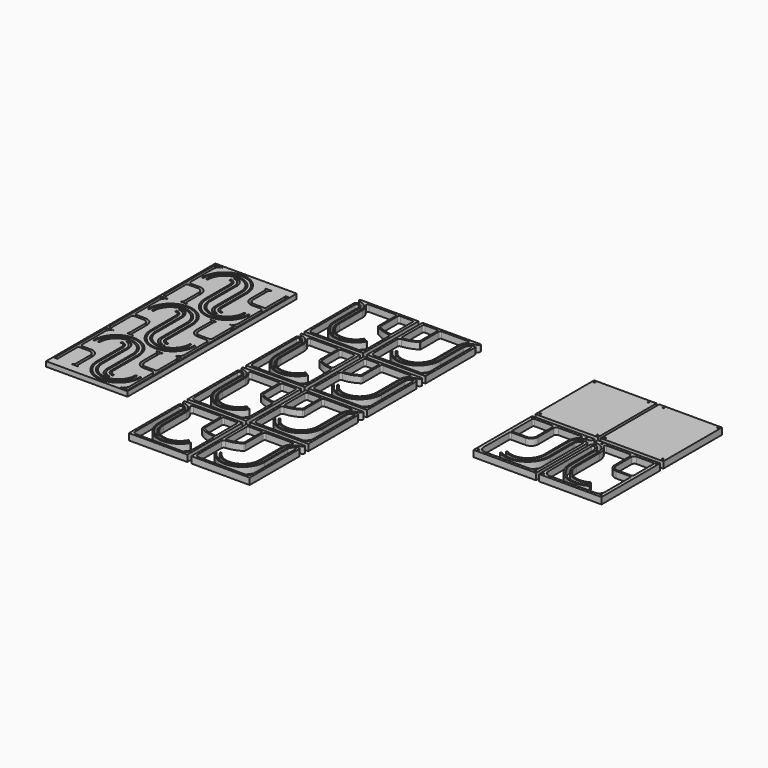
from build123d import *

# Parameters (mm, degrees)
F0_W     = 300
F0_H     = 780
F1_DEPTH = 18
F2_R     = 3
F3_DEPTH = 24
F2_W     = 230
F2_H     = 270
F2_W_2   = 231.0000000001
F5_DEPTH = 24


# Not quite as in the source:
# - a pattern or mirror of a feature is missing from the dataset's text; its kind, count and spacing are read off the source's solid


with BuildPart() as f1:
    # F0 (on Top) → F1 (new body)
    with BuildSketch(Plane.XY):
        with Locations((-546.0000000001, 50)):
            Rectangle(F0_W, F0_H)
        with BuildLine():
            Line((-690, -68), (-660, -68))
            ThreePointArc((-660, -68), (-674.1421356237, -73.8578643763), (-680, -88))
            Line((-680, -88), (-680, -192))
            ThreePointArc((-680, -192), (-677.0710678119, -199.0710678119), (-670, -202))
            Line((-670, -202), (-640, -202))
            ThreePointArc((-640, -202), (-618.7867965644, -210.7867965644), (-610, -232))
            Line((-610, -232), (-610, -298))
            ThreePointArc((-610, -298), (-607.0710678119, -305.0710678119), (-600, -308))
            Line((-600, -308), (-630, -308))
            ThreePointArc((-630, -308), (-622.9289321881, -305.0710678119), (-620, -298))
            Line((-620, -298), (-620, -232))
            ThreePointArc((-620, -232), (-625.8578643763, -217.8578643763), (-640, -212))
            Line((-640, -212), (-675, -212))
            ThreePointArc((-675, -212), (-678.5355339059, -213.4644660941), (-680, -217))
            Line((-680, -217), (-680, -303))
            ThreePointArc((-680, -303), (-678.5355339059, -306.5355339059), (-675, -308))
            Line((-675, -308), (-690, -308))
            Line((-690, -308), (-690, -68))
        make_face(mode=Mode.SUBTRACT)
        with BuildLine():
            ThreePointArc((-490, -290), (-506.9705627485, -282.9705627485), (-514, -266))
            Line((-514, -266), (-514, -150))
            ThreePointArc((-514, -150), (-590, -74), (-666, -150))
            ThreePointArc((-666, -150), (-669, -153), (-672, -150))
            ThreePointArc((-672, -150), (-590, -68), (-508, -150))
            Line((-508, -150), (-508, -266))
            ThreePointArc((-508, -266), (-502.7279220614, -278.7279220614), (-490, -284))
            Line((-490, -284), (-490, -290))
        make_face(mode=Mode.SUBTRACT)
        with BuildLine():
            ThreePointArc((-515, -300), (-526.6880815177, -284.8476830225), (-530, -266))
            Line((-530, -266), (-530, -150))
            ThreePointArc((-530, -150), (-590, -90), (-650, -150))
            ThreePointArc((-650, -150), (-653, -153), (-656, -150))
            ThreePointArc((-656, -150), (-590, -84), (-524, -150))
            Line((-524, -150), (-524, -266))
            ThreePointArc((-524, -266), (-514.0416305603, -290.0416305603), (-490, -300))
            Line((-490, -300), (-515, -300))
        make_face(mode=Mode.SUBTRACT)
        with BuildLine():
            ThreePointArc((-600, -110), (-583.0294372515, -117.0294372515), (-576, -134))
            Line((-576, -134), (-576, -250))
            ThreePointArc((-576, -250), (-500, -326), (-424, -250))
            ThreePointArc((-424, -250), (-421, -247), (-418, -250))
            ThreePointArc((-418, -250), (-500, -332), (-582, -250))
            Line((-582, -250), (-582, -134))
            ThreePointArc((-582, -134), (-587.2720779386, -121.2720779386), (-600, -116))
            Line((-600, -116), (-600, -110))
        make_face(mode=Mode.SUBTRACT)
        with BuildLine():
            ThreePointArc((-575, -100), (-563.3119184823, -115.1523169775), (-560, -134))
            Line((-560, -134), (-560, -250))
            ThreePointArc((-560, -250), (-500, -310), (-440, -250))
            ThreePointArc((-440, -250), (-437, -247), (-434, -250))
            ThreePointArc((-434, -250), (-500, -316), (-566, -250))
            Line((-566, -250), (-566, -134))
            ThreePointArc((-566, -134), (-575.9583694397, -109.9583694397), (-600, -100))
            Line((-600, -100), (-575, -100))
        make_face(mode=Mode.SUBTRACT)
        with BuildLine():
            Line((-400, -332), (-430, -332))
            ThreePointArc((-430, -332), (-415.8578643763, -326.1421356237), (-410, -312))
            Line((-410, -312), (-410, -208))
            ThreePointArc((-410, -208), (-412.9289321881, -200.9289321881), (-420, -198))
            Line((-420, -198), (-450, -198))
            ThreePointArc((-450, -198), (-471.2132034356, -189.2132034356), (-480, -168))
            Line((-480, -168), (-480, -102))
            ThreePointArc((-480, -102), (-482.9289321881, -94.9289321881), (-490, -92))
            Line((-490, -92), (-460, -92))
            ThreePointArc((-460, -92), (-467.0710678119, -94.9289321881), (-470, -102))
            Line((-470, -102), (-470, -168))
            ThreePointArc((-470, -168), (-464.1421356237, -182.1421356237), (-450, -188))
            Line((-450, -188), (-415, -188))
            ThreePointArc((-415, -188), (-411.4644660941, -186.5355339059), (-410, -183))
            Line((-410, -183), (-410, -97))
            ThreePointArc((-410, -97), (-411.4644660941, -93.4644660941), (-415, -92))
            Line((-415, -92), (-400, -92))
            Line((-400, -92), (-400, -332))
        make_face(mode=Mode.SUBTRACT)
        with BuildLine():
            ThreePointArc((-600, 140), (-583.0294372515, 132.9705627485), (-576, 116))
            Line((-576, 116), (-576, 0))
            ThreePointArc((-576, 0), (-500, -76), (-424, 0))
            ThreePointArc((-424, 0), (-421, 3), (-418, 0))
            ThreePointArc((-418, 0), (-500, -82), (-582, 0))
            Line((-582, 0), (-582, 116))
            ThreePointArc((-582, 116), (-587.2720779386, 128.7279220614), (-600, 134))
            Line((-600, 134), (-600, 140))
        make_face(mode=Mode.SUBTRACT)
        with BuildLine():
            ThreePointArc((-575, 150), (-563.3119184823, 134.8476830225), (-560, 116))
            Line((-560, 116), (-560, 0))
            ThreePointArc((-560, 0), (-500, -60), (-440, 0))
            ThreePointArc((-440, 0), (-437, 3), (-434, 0))
            ThreePointArc((-434, 0), (-500, -66), (-566, 0))
            Line((-566, 0), (-566, 116))
            ThreePointArc((-566, 116), (-575.9583694397, 140.0416305603), (-600, 150))
            Line((-600, 150), (-575, 150))
        make_face(mode=Mode.SUBTRACT)
        with BuildLine():
            Line((-400, -82), (-430, -82))
            ThreePointArc((-430, -82), (-415.8578643763, -76.1421356237), (-410, -62))
            Line((-410, -62), (-410, 42))
            ThreePointArc((-410, 42), (-412.9289321881, 49.0710678119), (-420, 52))
            Line((-420, 52), (-450, 52))
            ThreePointArc((-450, 52), (-471.2132034356, 60.7867965644), (-480, 82))
            Line((-480, 82), (-480, 148))
            ThreePointArc((-480, 148), (-482.9289321881, 155.0710678119), (-490, 158))
            Line((-490, 158), (-460, 158))
            ThreePointArc((-460, 158), (-467.0710678119, 155.0710678119), (-470, 148))
            Line((-470, 148), (-470, 82))
            ThreePointArc((-470, 82), (-464.1421356237, 67.8578643763), (-450, 62))
            Line((-450, 62), (-415, 62))
            ThreePointArc((-415, 62), (-411.4644660941, 63.4644660941), (-410, 67))
            Line((-410, 67), (-410, 153))
            ThreePointArc((-410, 153), (-411.4644660941, 156.5355339059), (-415, 158))
            Line((-415, 158), (-400, 158))
            Line((-400, 158), (-400, -82))
        make_face(mode=Mode.SUBTRACT)
        with BuildLine():
            Line((-690.0000015681, 182.000000209), (-660.0000015681, 182.000000209))
            ThreePointArc((-660.0000015681, 182.000000209), (-674.1421371918, 176.1421358327), (-680.0000015681, 162.000000209))
            Line((-680.0000015681, 162.000000209), (-680.0000015681, 58.000000209))
            ThreePointArc((-680.0000015681, 58.000000209), (-677.07106938, 50.9289323971), (-670.0000015681, 48.000000209))
            Line((-670.0000015681, 48.000000209), (-640.0000015681, 48))
            ThreePointArc((-640.0000015681, 48), (-618.7867971188, 39.21320399), (-610, 18))
            Line((-610, 18), (-610, -48))
            ThreePointArc((-610, -48), (-607.0710678119, -55.0710678119), (-600, -58))
            Line((-600, -58), (-630, -58))
            ThreePointArc((-630, -58), (-622.9289321881, -55.0710678119), (-620, -48))
            Line((-620, -48), (-620, 18))
            ThreePointArc((-620, 18), (-625.8578649305, 32.1421361779), (-640.0000015674, 38))
            Line((-640.0000015674, 38), (-675.0000015674, 38.0000002439))
            ThreePointArc((-675.0000015674, 38.0000002439), (-678.5355354738, 36.53553415), (-680.0000015681, 33.0000002439))
            Line((-680.0000015681, 33.0000002439), (-680.0000015681, -52.9999997561))
            ThreePointArc((-680.0000015681, -52.9999997561), (-678.535535474, -56.5355336621), (-675.0000015681, -57.9999997561))
            Line((-675.0000015681, -57.9999997561), (-690.0000015681, -58))
            Line((-690.0000015681, -58), (-690.0000015681, 182.000000209))
        make_face(mode=Mode.SUBTRACT)
        with BuildLine():
            ThreePointArc((-490, -40), (-506.9705627485, -32.9705627485), (-514, -16))
            Line((-514, -16), (-514, 100))
            ThreePointArc((-514, 100), (-590, 176), (-666, 100))
            ThreePointArc((-666, 100), (-669, 97), (-672, 100))
            ThreePointArc((-672, 100), (-590, 182), (-508, 100))
            Line((-508, 100), (-508, -16))
            ThreePointArc((-508, -16), (-502.7279220614, -28.7279220614), (-490, -34))
            Line((-490, -34), (-490, -40))
        make_face(mode=Mode.SUBTRACT)
        with BuildLine():
            ThreePointArc((-515, -50), (-526.6880815177, -34.8476830225), (-530, -16))
            Line((-530, -16), (-530, 100))
            ThreePointArc((-530, 100), (-590, 160), (-650, 100))
            ThreePointArc((-650, 100), (-653, 97), (-656, 100))
            ThreePointArc((-656, 100), (-590, 166), (-524, 100))
            Line((-524, 100), (-524, -16))
            ThreePointArc((-524, -16), (-514.0416305603, -40.0416305603), (-490, -50))
            Line((-490, -50), (-515, -50))
        make_face(mode=Mode.SUBTRACT)
        with BuildLine():
            Line((-690.0000000001, 432), (-660.0000000001, 432))
            ThreePointArc((-660.0000000001, 432), (-674.1421356238, 426.1421356237), (-680.0000000001, 412))
            Line((-680.0000000001, 412), (-680.0000000001, 308))
            ThreePointArc((-680.0000000001, 308), (-677.071067812, 300.9289321881), (-670.0000000001, 298))
            Line((-670.0000000001, 298), (-640.0000000001, 298))
            ThreePointArc((-640.0000000001, 298), (-618.7867965646, 289.2132034356), (-610.0000000001, 268))
            Line((-610.0000000001, 268), (-610.0000000002, 202))
            ThreePointArc((-610.0000000002, 202), (-607.0710678121, 194.9289321881), (-600.0000000002, 192))
            Line((-600.0000000002, 192), (-630.0000000002, 192))
            ThreePointArc((-630.0000000002, 192), (-622.9289321883, 194.9289321881), (-620.0000000002, 202))
            Line((-620.0000000002, 202), (-620.0000000001, 268))
            ThreePointArc((-620.0000000001, 268), (-625.8578643764, 282.1421356237), (-640.0000000001, 288))
            Line((-640.0000000001, 288), (-675.0000000001, 288))
            ThreePointArc((-675.0000000001, 288), (-678.535533906, 286.5355339059), (-680.0000000001, 283))
            Line((-680.0000000001, 283), (-680.0000000001, 197))
            ThreePointArc((-680.0000000001, 197), (-678.5355339061, 193.464466094), (-675.0000000001, 192))
            Line((-675.0000000001, 192), (-690.0000000001, 192))
            Line((-690.0000000001, 192), (-690.0000000001, 432))
        make_face(mode=Mode.SUBTRACT)
        with BuildLine():
            ThreePointArc((-515, 200), (-526.6880815177, 215.1523169775), (-530, 234))
            Line((-530, 234), (-530, 350))
            ThreePointArc((-530, 350), (-590, 410), (-650, 350))
            ThreePointArc((-650, 350), (-653, 347), (-656, 350))
            ThreePointArc((-656, 350), (-590, 416), (-524, 350))
            Line((-524, 350), (-524, 234))
            ThreePointArc((-524, 234), (-514.0416305603, 209.9583694397), (-490, 200))
            Line((-490, 200), (-515, 200))
        make_face(mode=Mode.SUBTRACT)
        with BuildLine():
            ThreePointArc((-490, 210), (-506.9705627485, 217.0294372515), (-514, 234))
            Line((-514, 234), (-514, 350))
            ThreePointArc((-514, 350), (-590, 426), (-666, 350))
            ThreePointArc((-666, 350), (-669, 347), (-672, 350))
            ThreePointArc((-672, 350), (-590, 432), (-508, 350))
            Line((-508, 350), (-508, 234))
            ThreePointArc((-508, 234), (-502.7279220613, 221.2720779387), (-490, 216))
            Line((-490, 216), (-490, 210))
        make_face(mode=Mode.SUBTRACT)
        with BuildLine():
            ThreePointArc((-600, 390), (-583.0294372515, 382.9705627485), (-576, 366))
            Line((-576, 366), (-576, 250))
            ThreePointArc((-576, 250), (-500, 174), (-424, 250))
            ThreePointArc((-424, 250), (-421, 253), (-418, 250))
            ThreePointArc((-418, 250), (-500, 168), (-582, 250))
            Line((-582, 250), (-582, 366))
            ThreePointArc((-582, 366), (-587.2720779386, 378.7279220614), (-600, 384))
            Line((-600, 384), (-600, 390))
        make_face(mode=Mode.SUBTRACT)
        with BuildLine():
            ThreePointArc((-575, 400), (-563.3119184823, 384.8476830225), (-560, 366))
            Line((-560, 366), (-560, 250))
            ThreePointArc((-560, 250), (-500, 190), (-440, 250))
            ThreePointArc((-440, 250), (-437, 253), (-434, 250))
            ThreePointArc((-434, 250), (-500, 184), (-566, 250))
            Line((-566, 250), (-566, 366))
            ThreePointArc((-566, 366), (-575.9583694397, 390.0416305603), (-600, 400))
            Line((-600, 400), (-575, 400))
        make_face(mode=Mode.SUBTRACT)
        with BuildLine():
            Line((-400, 168), (-430, 168))
            ThreePointArc((-430, 168), (-415.8578643763, 173.8578643763), (-410, 188))
            Line((-410, 188), (-410, 292))
            ThreePointArc((-410, 292), (-412.9289321881, 299.0710678119), (-420, 302))
            Line((-420, 302), (-450, 302))
            ThreePointArc((-450, 302), (-471.2132034356, 310.7867965644), (-480, 332))
            Line((-480, 332), (-480, 398))
            ThreePointArc((-480, 398), (-482.9289321881, 405.0710678119), (-490, 408))
            Line((-490, 408), (-460, 408))
            ThreePointArc((-460, 408), (-467.0710678119, 405.0710678119), (-470, 398))
            Line((-470, 398), (-470, 332))
            ThreePointArc((-470, 332), (-464.1421356237, 317.8578643763), (-450, 312))
            Line((-450, 312), (-415, 312))
            ThreePointArc((-415, 312), (-411.4644660941, 313.4644660941), (-410, 317))
            Line((-410, 317), (-410, 403))
            ThreePointArc((-410, 403), (-411.4644660941, 406.5355339059), (-415, 408))
            Line((-415, 408), (-400, 408))
            Line((-400, 408), (-400, 168))
        make_face(mode=Mode.SUBTRACT)
    extrude(amount=F1_DEPTH)


with BuildPart() as f3:
    # F2 (on Top) → F3 (new body)
    with BuildSketch(Plane.XY):
        with BuildLine():
            Line((817.5872366072, -1.8937941178), (649.5872366071, -1.8937941178))
            ThreePointArc((649.5872366071, -1.8937941178), (635.4451009834, 3.9640702585), (629.5872366071, 18.1062058822))
            Line((629.5872366071, 18.1062058822), (629.5872366071, 136.1062058824))
            ThreePointArc((629.5872366071, 136.1062058824), (631.0517027012, 139.6417397883), (634.5872366071, 141.1062058824))
            Line((634.5872366071, 141.1062058824), (686.5872366071, 141.1062058824))
            ThreePointArc((686.5872366071, 141.1062058824), (704.972012918, 148.7214295715), (712.5872366071, 167.1062058824))
            Line((712.5872366071, 167.1062058824), (712.5872366071, 238.1062058824))
            ThreePointArc((712.5872366071, 238.1062058824), (715.5161687953, 245.1772736942), (722.5872366071, 248.1062058824))
            Line((722.5872366071, 248.1062058824), (807.5872366073, 248.1062058824))
            ThreePointArc((807.5872366073, 248.1062058824), (811.9651765489, 245.5214992119), (811.8168402625, 240.4396626294))
            ThreePointArc((811.8168402625, 240.4396626294), (798.4656500559, 222.1876642916), (793.5872366072, 200.1062058824))
            Line((793.5872366072, 200.1062058824), (793.5872366072, 93.1062058822))
            ThreePointArc((793.5872366072, 93.1062058822), (763.0872366072, 40.2786562514), (702.0872366072, 40.2786562514))
            ThreePointArc((702.0872366072, 40.2786562514), (697.9891603959, 39.18058004), (699.0872366072, 35.0825038287))
            ThreePointArc((699.0872366072, 35.0825038287), (766.0872366072, 35.0825038287), (799.5872366072, 93.1062058822))
            Line((799.5872366072, 93.1062058822), (799.5872366072, 200.1062058824))
            ThreePointArc((799.5872366072, 200.1062058824), (810.4624797989, 228.6894177383), (837.5872366074, 242.8145188905))
            ThreePointArc((837.5872366074, 242.8145188905), (844.7634629803, 245.8458146212), (847.5872366072, 253.1062058824))
            Line((847.5872366072, 253.1062058824), (847.5872366071, 258.1062058824))
            Line((847.5872366071, 258.1062058824), (617.5872366071, 258.1062058824))
            Line((617.5872366071, 258.1062058824), (617.5872366071, -11.8937941178))
            Line((617.5872366071, -11.8937941178), (847.5872366072, -11.8937941178))
            Line((847.5872366072, -11.8937941178), (847.5872366072, 221.1062058824))
            ThreePointArc((847.5872366072, 221.1062058824), (843.778224948, 228.3850749319), (835.8025559711, 230.3546456548))
            ThreePointArc((835.8025559711, 230.3546456548), (818.3867707055, 219.4798335793), (811.5872366072, 200.1062058824))
            Line((811.5872366072, 200.1062058824), (811.5872366072, 93.1062058822))
            ThreePointArc((811.5872366072, 93.1062058822), (772.0872366072, 24.6901989832), (693.0872366072, 24.6901989832))
            ThreePointArc((693.0872366072, 24.6901989832), (688.9891603959, 23.5921227719), (690.0872366072, 19.4940465605))
            ThreePointArc((690.0872366072, 19.4940465605), (775.0872366072, 19.4940465605), (817.5872366072, 93.1062058822))
            Line((817.5872366072, 93.1062058822), (817.5872366072, 200.1062058824))
            ThreePointArc((817.5872366072, 200.1062058824), (821.0893760407, 212.8671616092), (830.6145958922, 222.0528656352))
            ThreePointArc((830.6145958922, 222.0528656352), (835.2778681125, 221.6750699203), (837.5872366072, 217.6062058824))
            Line((837.5872366072, 217.6062058824), (837.5872366072, 18.1062058822))
            ThreePointArc((837.5872366072, 18.1062058822), (831.729372231, 3.9640702585), (817.5872366072, -1.8937941178))
        make_face()
        with Locations((627.5872366071, -1.8937941178)):
            Circle(F2_R, mode=Mode.SUBTRACT)
        with Locations((838.5872366072, -2.8937941178)):
            Circle(F2_R, mode=Mode.SUBTRACT)
        with BuildLine():
            Line((686.5872366071, 147.1062058824), (634.5872366071, 147.1062058824))
            ThreePointArc((634.5872366071, 147.1062058824), (631.0517027012, 148.5706719765), (629.5872366071, 152.1062058824))
            Line((629.5872366071, 152.1062058824), (629.5872366071, 243.1062058824))
            ThreePointArc((629.5872366071, 243.1062058824), (631.0517027012, 246.6417397883), (634.5872366071, 248.1062058824))
            Line((634.5872366071, 248.1062058824), (696.5872366071, 248.1062058824))
            ThreePointArc((696.5872366071, 248.1062058824), (703.658304419, 245.1772736942), (706.5872366071, 238.1062058824))
            Line((706.5872366071, 238.1062058824), (706.5872366071, 167.1062058824))
            ThreePointArc((706.5872366071, 167.1062058824), (700.7293722309, 152.9640702587), (686.5872366071, 147.1062058824))
        make_face(mode=Mode.SUBTRACT)
        with Locations((625.0872366071, 250.6062058824)):
            Circle(F2_R, mode=Mode.SUBTRACT)
        with Locations((824.5872366073, 249.1062058824)):
            Circle(F2_R, mode=Mode.SUBTRACT)
    extrude(amount=F3_DEPTH)


with BuildPart() as f3b:
    # F2 (on Top) → F3, piece 2 (new body)
    with BuildSketch(Plane.XY):
        with Locations((732.5872366071, 408.5740244389)):
            Rectangle(F2_W, F2_H)
        with Locations((627.5872366071, 283.5740244389)):
            Circle(F2_R, mode=Mode.SUBTRACT)
        with Locations((838.5872366071, 282.5740244389)):
            Circle(F2_R, mode=Mode.SUBTRACT)
        with Locations((625.0872366071, 536.0740244389)):
            Circle(F2_R, mode=Mode.SUBTRACT)
        with Locations((824.5872366071, 534.5740244389)):
            Circle(F2_R, mode=Mode.SUBTRACT)
    extrude(amount=F3_DEPTH)


with BuildPart() as f3c:
    # F2 (on Top) → F3, piece 3 (new body)
    with BuildSketch(Plane.XY):
        with Locations((973.0872366074, 408.5740244389)):
            Rectangle(F2_W_2, F2_H)
        with Locations((866.5872366073, 282.5740244389)):
            Circle(F2_R, mode=Mode.SUBTRACT)
        with Locations((1078.5872366074, 283.5740244389)):
            Circle(F2_R, mode=Mode.SUBTRACT)
        with Locations((880.5872366073, 534.5740244389)):
            Circle(F2_R, mode=Mode.SUBTRACT)
        with Locations((1081.0872366074, 536.0740244389)):
            Circle(F2_R, mode=Mode.SUBTRACT)
    extrude(amount=F3_DEPTH)


with BuildPart() as f3d:
    # F2 (on Top) → F3, piece 4 (new body)
    with BuildSketch(Plane.XY):
        with BuildLine():
            Line((1088.9746864199, -11.8937941178), (1088.9746864199, 258.1062058824))
            Line((1088.9746864199, 258.1062058824), (858.9746864199, 258.1062058824))
            Line((858.9746864199, 258.1062058824), (858.9746864198, 253.1062058824))
            ThreePointArc((858.9746864198, 253.1062058824), (861.7984600468, 245.8458146212), (868.9746864197, 242.8145188905))
            ThreePointArc((868.9746864197, 242.8145188905), (896.0994432282, 228.6894177383), (906.9746864198, 200.1062058824))
            Line((906.9746864198, 200.1062058824), (906.9746864198, 93.1062058822))
            ThreePointArc((906.9746864198, 93.1062058822), (940.4746864198, 35.0825038287), (1007.4746864198, 35.0825038287))
            ThreePointArc((1007.4746864198, 35.0825038287), (1008.5727626312, 39.18058004), (1004.4746864198, 40.2786562514))
            ThreePointArc((1004.4746864198, 40.2786562514), (943.4746864198, 40.2786562514), (912.9746864198, 93.1062058822))
            Line((912.9746864198, 93.1062058822), (912.9746864198, 200.1062058824))
            ThreePointArc((912.9746864198, 200.1062058824), (908.0962729712, 222.1876642916), (894.7450827646, 240.4396626294))
            ThreePointArc((894.7450827646, 240.4396626294), (894.5967464781, 245.5214992119), (898.9746864197, 248.1062058824))
            Line((898.9746864197, 248.1062058824), (983.9746864199, 248.1062058824))
            ThreePointArc((983.9746864199, 248.1062058824), (991.0457542318, 245.1772736942), (993.9746864199, 238.1062058824))
            Line((993.9746864199, 238.1062058824), (993.9746864199, 167.1062058824))
            ThreePointArc((993.9746864199, 167.1062058824), (1001.589910109, 148.7214295715), (1019.9746864199, 141.1062058824))
            Line((1019.9746864199, 141.1062058824), (1071.9746864199, 141.1062058824))
            ThreePointArc((1071.9746864199, 141.1062058824), (1075.5102203258, 139.6417397883), (1076.9746864199, 136.1062058824))
            Line((1076.9746864199, 136.1062058824), (1076.9746864199, 18.1062058822))
            ThreePointArc((1076.9746864199, 18.1062058822), (1071.1168220436, 3.9640702585), (1056.9746864199, -1.8937941178))
            Line((1056.9746864199, -1.8937941178), (888.9746864198, -1.8937941178))
            ThreePointArc((888.9746864198, -1.8937941178), (874.8325507961, 3.9640702585), (868.9746864198, 18.1062058822))
            Line((868.9746864198, 18.1062058822), (868.9746864198, 217.6062058824))
            ThreePointArc((868.9746864198, 217.6062058824), (871.2840549145, 221.6750699203), (875.9473271349, 222.0528656352))
            ThreePointArc((875.9473271349, 222.0528656352), (885.4725469864, 212.8671616092), (888.9746864198, 200.1062058824))
            Line((888.9746864198, 200.1062058824), (888.9746864198, 93.1062058822))
            ThreePointArc((888.9746864198, 93.1062058822), (931.4746864198, 19.4940465605), (1016.4746864198, 19.4940465605))
            ThreePointArc((1016.4746864198, 19.4940465605), (1017.5727626312, 23.5921227719), (1013.4746864198, 24.6901989832))
            ThreePointArc((1013.4746864198, 24.6901989832), (934.4746864198, 24.6901989832), (894.9746864198, 93.1062058822))
            Line((894.9746864198, 93.1062058822), (894.9746864198, 200.1062058824))
            ThreePointArc((894.9746864198, 200.1062058824), (888.1751523215, 219.4798335793), (870.7593670559, 230.3546456548))
            ThreePointArc((870.7593670559, 230.3546456548), (862.7836980791, 228.3850749319), (858.9746864198, 221.1062058824))
            Line((858.9746864198, 221.1062058824), (858.9746864198, -11.8937941178))
            Line((858.9746864198, -11.8937941178), (1088.9746864199, -11.8937941178))
        make_face()
        with Locations((867.9746864198, -2.8937941178)):
            Circle(F2_R, mode=Mode.SUBTRACT)
        with Locations((1078.9746864199, -1.8937941178)):
            Circle(F2_R, mode=Mode.SUBTRACT)
        with Locations((881.9746864198, 249.1062058824)):
            Circle(F2_R, mode=Mode.SUBTRACT)
        with BuildLine():
            ThreePointArc((1076.9746864199, 152.1062058824), (1075.5102203258, 148.5706719765), (1071.9746864199, 147.1062058824))
            Line((1071.9746864199, 147.1062058824), (1019.9746864199, 147.1062058824))
            ThreePointArc((1019.9746864199, 147.1062058824), (1005.8325507962, 152.9640702587), (999.9746864199, 167.1062058824))
            Line((999.9746864199, 167.1062058824), (999.9746864199, 238.1062058824))
            ThreePointArc((999.9746864199, 238.1062058824), (1002.903618608, 245.1772736942), (1009.9746864199, 248.1062058824))
            Line((1009.9746864199, 248.1062058824), (1071.9746864199, 248.1062058824))
            ThreePointArc((1071.9746864199, 248.1062058824), (1075.5102203258, 246.6417397883), (1076.9746864199, 243.1062058824))
            Line((1076.9746864199, 243.1062058824), (1076.9746864199, 152.1062058824))
        make_face(mode=Mode.SUBTRACT)
        with Locations((1081.4746864199, 250.6062058824)):
            Circle(F2_R, mode=Mode.SUBTRACT)
    extrude(amount=F3_DEPTH)


with BuildPart() as f5:
    # F4 (on Top) → F5 (new body)
    with BuildSketch(Plane.XY):
        with BuildLine():
            Line((202.0814875615, -542), (28, -542))
            ThreePointArc((28, -542), (19.1611652352, -538.3388347648), (15.5, -529.5))
            Line((15.5, -529.5), (15.5, -420.7087052152))
            ThreePointArc((15.5, -420.7087052152), (17.8431457505, -415.0518509657), (23.5, -412.7087052152))
            ThreePointArc((23.5, -412.7087052152), (51.5368274071, -406.9295293477), (77.1330902678, -394.1118114409))
            ThreePointArc((77.1330902678, -394.1118114409), (78.5035898285, -391.717491115), (78.9792797578, -389))
            Line((78.9792797578, -389), (78.9792797578, -309))
            ThreePointArc((78.9792797578, -309), (80.7366390707, -304.7573593129), (84.9792797578, -303))
            Line((84.9792797578, -303), (182.8439484799, -303))
            ThreePointArc((182.8439484799, -303), (188.06860498, -306.0499212796), (187.9816644673, -312.0990118478))
            ThreePointArc((187.9816644673, -312.0990118478), (179.0054808002, -325.8532418068), (176, -342))
            Line((176, -342), (176, -448))
            ThreePointArc((176, -448), (130.7879617513, -506.9214754036), (62.1724503691, -478.5))
            ThreePointArc((62.1724503691, -478.5), (58.7573868597, -477.5849364905), (57.8423233502, -481))
            ThreePointArc((57.8423233502, -481), (132.0820569768, -511.7511045351), (181, -448))
            Line((181, -448), (181, -342))
            ThreePointArc((181, -342), (190.6508845583, -317.2740015368), (214.5, -305.6234965946))
            ThreePointArc((214.5, -305.6234965946), (220.1568542495, -303.2803508441), (222.5, -297.6234965946))
            Line((222.5, -297.6234965946), (222.5, -295))
            Line((222.5, -295), (7.5, -295))
            Line((7.5, -295), (7.5, -550))
            Line((7.5, -550), (222.5, -550))
            Line((222.5, -550), (222.5, -323.2359864067))
            ThreePointArc((222.5, -323.2359864067), (219.7780031628, -317.224107947), (213.4643293466, -315.3033080256))
            ThreePointArc((213.4643293466, -315.3033080256), (197.0309610919, -324.3926593099), (190.5, -342))
            Line((190.5, -342), (190.5, -448))
            ThreePointArc((190.5, -448), (134.5408379052, -520.9273998848), (49.6150820143, -485.75))
            ThreePointArc((49.6150820143, -485.75), (46.2000185048, -484.8349364905), (45.2849549954, -488.25))
            ThreePointArc((45.2849549954, -488.25), (135.8349331308, -525.7570290163), (195.5, -448))
            Line((195.5, -448), (195.5, -342))
            ThreePointArc((195.5, -342), (197.9851168632, -331.8427692673), (204.8790305598, -323.9802572052))
            ThreePointArc((204.8790305598, -323.9802572052), (211.171533582, -323.3920372351), (214.5, -328.7644583207))
            Line((214.5, -328.7644583207), (214.5814875615, -529.5))
            ThreePointArc((214.5814875615, -529.5), (210.9203223264, -538.3388347648), (202.0814875615, -542))
        make_face()
        with BuildLine():
            ThreePointArc((23.5, -406.7087052152), (19.2573593129, -404.9513459023), (17.5, -400.7087052152))
            Line((17.5, -400.7087052152), (17.5, -309))
            ThreePointArc((17.5, -309), (19.2573593129, -304.7573593129), (23.5, -303))
            Line((23.5, -303), (66.9792797578, -303))
            ThreePointArc((66.9792797578, -303), (71.2219204449, -304.7573593129), (72.9792797578, -309))
            Line((72.9792797578, -309), (72.9792797578, -386.5))
            ThreePointArc((72.9792797578, -386.5), (72.4414458031, -388.9828898674), (70.9243657265, -391.0206522427))
            ThreePointArc((70.9243657265, -391.0206522427), (48.1678939246, -401.7537555941), (23.5, -406.7087052152))
        make_face(mode=Mode.SUBTRACT)
    extrude(amount=F5_DEPTH)


with BuildPart() as f5b:
    # F4 (on Top) → F5, piece 2 (new body)
    with BuildSketch(Plane.XY):
        with BuildLine():
            Line((7.5, -25), (7.5, -280))
            Line((7.5, -280), (222.5, -280))
            Line((222.5, -280), (222.5, -53.2359864067))
            ThreePointArc((222.5, -53.2359864067), (219.7780031628, -47.224107947), (213.4643293466, -45.3033080256))
            ThreePointArc((213.4643293466, -45.3033080256), (197.0309610919, -54.3926593099), (190.5, -72))
            Line((190.5, -72), (190.5, -178))
            ThreePointArc((190.5, -178), (134.5408379052, -250.9273998848), (49.6150820143, -215.75))
            ThreePointArc((49.6150820143, -215.75), (46.2000185048, -214.8349364905), (45.2849549954, -218.25))
            ThreePointArc((45.2849549954, -218.25), (135.8349331308, -255.7570290163), (195.5, -178))
            Line((195.5, -178), (195.5, -72))
            ThreePointArc((195.5, -72), (197.9851168632, -61.8427692673), (204.8790305598, -53.9802572052))
            ThreePointArc((204.8790305598, -53.9802572052), (211.171533582, -53.3920372351), (214.5, -58.7644583207))
            Line((214.5, -58.7644583207), (214.5814875615, -259.5))
            ThreePointArc((214.5814875615, -259.5), (210.9203223264, -268.3388347648), (202.0814875615, -272))
            Line((202.0814875615, -272), (28, -272))
            ThreePointArc((28, -272), (19.1611652352, -268.3388347648), (15.5, -259.5))
            Line((15.5, -259.5), (15.5, -150.7087052152))
            ThreePointArc((15.5, -150.7087052152), (17.8431457505, -145.0518509657), (23.5, -142.7087052152))
            ThreePointArc((23.5, -142.7087052152), (51.5368274071, -136.9295293477), (77.1330902678, -124.1118114409))
            ThreePointArc((77.1330902678, -124.1118114409), (78.5035898285, -121.717491115), (78.9792797578, -119))
            Line((78.9792797578, -119), (78.9792797578, -39))
            ThreePointArc((78.9792797578, -39), (80.7366390707, -34.7573593129), (84.9792797578, -33))
            Line((84.9792797578, -33), (182.8439484799, -33))
            ThreePointArc((182.8439484799, -33), (188.06860498, -36.0499212796), (187.9816644673, -42.0990118478))
            ThreePointArc((187.9816644673, -42.0990118478), (179.0054808002, -55.8532418068), (176, -72))
            Line((176, -72), (176, -178))
            ThreePointArc((176, -178), (130.7879617513, -236.9214754036), (62.1724503691, -208.5))
            ThreePointArc((62.1724503691, -208.5), (58.7573868597, -207.5849364905), (57.8423233502, -211))
            ThreePointArc((57.8423233502, -211), (132.0820569768, -241.7511045351), (181, -178))
            Line((181, -178), (181, -72))
            ThreePointArc((181, -72), (190.6508845583, -47.2740015368), (214.5, -35.6234965946))
            ThreePointArc((214.5, -35.6234965946), (220.1568542495, -33.2803508441), (222.5, -27.6234965946))
            Line((222.5, -27.6234965946), (222.5, -25))
            Line((222.5, -25), (7.5, -25))
        make_face()
        with BuildLine():
            ThreePointArc((17.5, -39), (19.2573593129, -34.7573593129), (23.5, -33))
            Line((23.5, -33), (66.9792797578, -33))
            ThreePointArc((66.9792797578, -33), (71.2219204449, -34.7573593129), (72.9792797578, -39))
            Line((72.9792797578, -39), (72.9792797578, -116.5))
            ThreePointArc((72.9792797578, -116.5), (72.4414458031, -118.9828898674), (70.9243657265, -121.0206522427))
            ThreePointArc((70.9243657265, -121.0206522427), (48.1678939246, -131.7537555941), (23.5, -136.7087052152))
            ThreePointArc((23.5, -136.7087052152), (19.2573593129, -134.9513459023), (17.5, -130.7087052152))
            Line((17.5, -130.7087052152), (17.5, -39))
        make_face(mode=Mode.SUBTRACT)
    extrude(amount=F5_DEPTH)


with BuildPart() as f5c:
    # F4 (on Top) → F5, piece 3 (new body)
    with BuildSketch(Plane.XY):
        with BuildLine():
            Line((7.5, 245), (7.5, -10))
            Line((7.5, -10), (222.5, -10))
            Line((222.5, -10), (222.5, 216.7640135933))
            ThreePointArc((222.5, 216.7640135933), (219.7780031628, 222.775892053), (213.4643293466, 224.6966919744))
            ThreePointArc((213.4643293466, 224.6966919744), (197.0309610919, 215.6073406901), (190.5, 198))
            Line((190.5, 198), (190.5, 92))
            ThreePointArc((190.5, 92), (134.5408379052, 19.0726001152), (49.6150820143, 54.25))
            ThreePointArc((49.6150820143, 54.25), (46.2000185048, 55.1650635095), (45.2849549954, 51.75))
            ThreePointArc((45.2849549954, 51.75), (135.8349331308, 14.2429709837), (195.5, 92))
            Line((195.5, 92), (195.5, 198))
            ThreePointArc((195.5, 198), (197.9851168632, 208.1572307327), (204.8790305598, 216.0197427948))
            ThreePointArc((204.8790305598, 216.0197427948), (211.171533582, 216.6079627649), (214.5, 211.2355416793))
            Line((214.5, 211.2355416793), (214.5814875615, 10.5))
            ThreePointArc((214.5814875615, 10.5), (210.9203223264, 1.6611652352), (202.0814875615, -2))
            Line((202.0814875615, -2), (28, -2))
            ThreePointArc((28, -2), (19.1611652352, 1.6611652352), (15.5, 10.5))
            Line((15.5, 10.5), (15.5, 119.2912947848))
            ThreePointArc((15.5, 119.2912947848), (17.8431457505, 124.9481490343), (23.5, 127.2912947848))
            ThreePointArc((23.5, 127.2912947848), (51.5368274071, 133.0704706523), (77.1330902678, 145.8881885591))
            ThreePointArc((77.1330902678, 145.8881885591), (78.5035898285, 148.282508885), (78.9792797578, 151))
            Line((78.9792797578, 151), (78.9792797578, 231))
            ThreePointArc((78.9792797578, 231), (80.7366390707, 235.2426406871), (84.9792797578, 237))
            Line((84.9792797578, 237), (182.8439484799, 237))
            ThreePointArc((182.8439484799, 237), (188.06860498, 233.9500787204), (187.9816644673, 227.9009881522))
            ThreePointArc((187.9816644673, 227.9009881522), (179.0054808002, 214.1467581932), (176, 198))
            Line((176, 198), (176, 92))
            ThreePointArc((176, 92), (130.7879617513, 33.0785245964), (62.1724503691, 61.5))
            ThreePointArc((62.1724503691, 61.5), (58.7573868597, 62.4150635095), (57.8423233502, 59))
            ThreePointArc((57.8423233502, 59), (132.0820569768, 28.2488954649), (181, 92))
            Line((181, 92), (181, 198))
            ThreePointArc((181, 198), (190.6508845583, 222.7259984632), (214.5, 234.3765034054))
            ThreePointArc((214.5, 234.3765034054), (220.1568542495, 236.7196491559), (222.5, 242.3765034054))
            Line((222.5, 242.3765034054), (222.5, 245))
            Line((222.5, 245), (7.5, 245))
        make_face()
        with BuildLine():
            ThreePointArc((17.5, 231), (19.2573593129, 235.2426406871), (23.5, 237))
            Line((23.5, 237), (66.9792797578, 237))
            ThreePointArc((66.9792797578, 237), (71.2219204449, 235.2426406871), (72.9792797578, 231))
            Line((72.9792797578, 231), (72.9792797578, 153.5))
            ThreePointArc((72.9792797578, 153.5), (72.4414458031, 151.0171101326), (70.9243657265, 148.9793477573))
            ThreePointArc((70.9243657265, 148.9793477573), (48.1678939246, 138.2462444059), (23.5, 133.2912947848))
            ThreePointArc((23.5, 133.2912947848), (19.2573593129, 135.0486540977), (17.5, 139.2912947848))
            Line((17.5, 139.2912947848), (17.5, 231))
        make_face(mode=Mode.SUBTRACT)
    extrude(amount=F5_DEPTH)


with BuildPart() as f5d:
    # F4 (on Top) → F5, piece 4 (new body)
    with BuildSketch(Plane.XY):
        with BuildLine():
            Line((7.5, 515), (7.5, 260))
            Line((7.5, 260), (222.5, 260))
            Line((222.5, 260), (222.5, 486.7640135933))
            ThreePointArc((222.5, 486.7640135933), (219.7780031628, 492.775892053), (213.4643293466, 494.6966919744))
            ThreePointArc((213.4643293466, 494.6966919744), (197.0309610919, 485.6073406901), (190.5, 468))
            Line((190.5, 468), (190.5, 362))
            ThreePointArc((190.5, 362), (134.5408379052, 289.0726001152), (49.6150820143, 324.25))
            ThreePointArc((49.6150820143, 324.25), (46.2000185048, 325.1650635095), (45.2849549954, 321.75))
            ThreePointArc((45.2849549954, 321.75), (135.8349331308, 284.2429709837), (195.5, 362))
            Line((195.5, 362), (195.5, 468))
            ThreePointArc((195.5, 468), (197.9851168632, 478.1572307327), (204.8790305598, 486.0197427948))
            ThreePointArc((204.8790305598, 486.0197427948), (211.171533582, 486.6079627649), (214.5, 481.2355416793))
            Line((214.5, 481.2355416793), (214.5814875615, 280.5))
            ThreePointArc((214.5814875615, 280.5), (210.9203223264, 271.6611652352), (202.0814875615, 268))
            Line((202.0814875615, 268), (28, 268))
            ThreePointArc((28, 268), (19.1611652352, 271.6611652352), (15.5, 280.5))
            Line((15.5, 280.5), (15.5, 389.2912947848))
            ThreePointArc((15.5, 389.2912947848), (17.8431457505, 394.9481490343), (23.5, 397.2912947848))
            ThreePointArc((23.5, 397.2912947848), (51.5368274071, 403.0704706523), (77.1330902678, 415.8881885591))
            ThreePointArc((77.1330902678, 415.8881885591), (78.5035898285, 418.282508885), (78.9792797578, 421))
            Line((78.9792797578, 421), (78.9792797578, 501))
            ThreePointArc((78.9792797578, 501), (80.7366390707, 505.2426406871), (84.9792797578, 507))
            Line((84.9792797578, 507), (182.8439484799, 507))
            ThreePointArc((182.8439484799, 507), (188.06860498, 503.9500787204), (187.9816644673, 497.9009881522))
            ThreePointArc((187.9816644673, 497.9009881522), (179.0054808002, 484.1467581932), (176, 468))
            Line((176, 468), (176, 362))
            ThreePointArc((176, 362), (130.7879617513, 303.0785245964), (62.1724503691, 331.5))
            ThreePointArc((62.1724503691, 331.5), (58.7573868597, 332.4150635095), (57.8423233502, 329))
            ThreePointArc((57.8423233502, 329), (132.0820569768, 298.2488954649), (181, 362))
            Line((181, 362), (181, 468))
            ThreePointArc((181, 468), (190.6508845583, 492.7259984632), (214.5, 504.3765034054))
            ThreePointArc((214.5, 504.3765034054), (220.1568542495, 506.7196491559), (222.5, 512.3765034054))
            Line((222.5, 512.3765034054), (222.5, 515))
            Line((222.5, 515), (7.5, 515))
        make_face()
        with BuildLine():
            ThreePointArc((17.5, 501), (19.2573593129, 505.2426406871), (23.5, 507))
            Line((23.5, 507), (66.9792797578, 507))
            ThreePointArc((66.9792797578, 507), (71.2219204449, 505.2426406871), (72.9792797578, 501))
            Line((72.9792797578, 501), (72.9792797578, 423.5))
            ThreePointArc((72.9792797578, 423.5), (72.4414458031, 421.0171101326), (70.9243657265, 418.9793477573))
            ThreePointArc((70.9243657265, 418.9793477573), (48.1678939246, 408.2462444059), (23.5, 403.2912947848))
            ThreePointArc((23.5, 403.2912947848), (19.2573593129, 405.0486540977), (17.5, 409.2912947848))
            Line((17.5, 409.2912947848), (17.5, 501))
        make_face(mode=Mode.SUBTRACT)
    extrude(amount=F5_DEPTH)


with BuildPart() as f5_copies_1:
    # F5_copies: instance of F5
    add(f5.part.mirror(Plane(origin=(0, 0, 0), x_dir=(0, 0, -1), z_dir=(-1, 0, 0))))


with BuildPart() as f5_2_copies_1:
    # F5_2_copies: instance of F5b
    add(f5b.part.mirror(Plane(origin=(0, 0, 0), x_dir=(0, 0, -1), z_dir=(-1, 0, 0))))


with BuildPart() as f5_3_copies_1:
    # F5_3_copies: instance of F5c
    add(f5c.part.mirror(Plane(origin=(0, 0, 0), x_dir=(0, 0, -1), z_dir=(-1, 0, 0))))


with BuildPart() as f5_4_copies_1:
    # F5_4_copies: instance of F5d
    add(f5d.part.mirror(Plane(origin=(0, 0, 0), x_dir=(0, 0, -1), z_dir=(-1, 0, 0))))


solid = Compound([f1.part, f3.part, f3b.part, f3c.part, f3d.part, f5.part, f5b.part, f5c.part, f5d.part, f5_copies_1.part, f5_2_copies_1.part, f5_3_copies_1.part, f5_4_copies_1.part])
